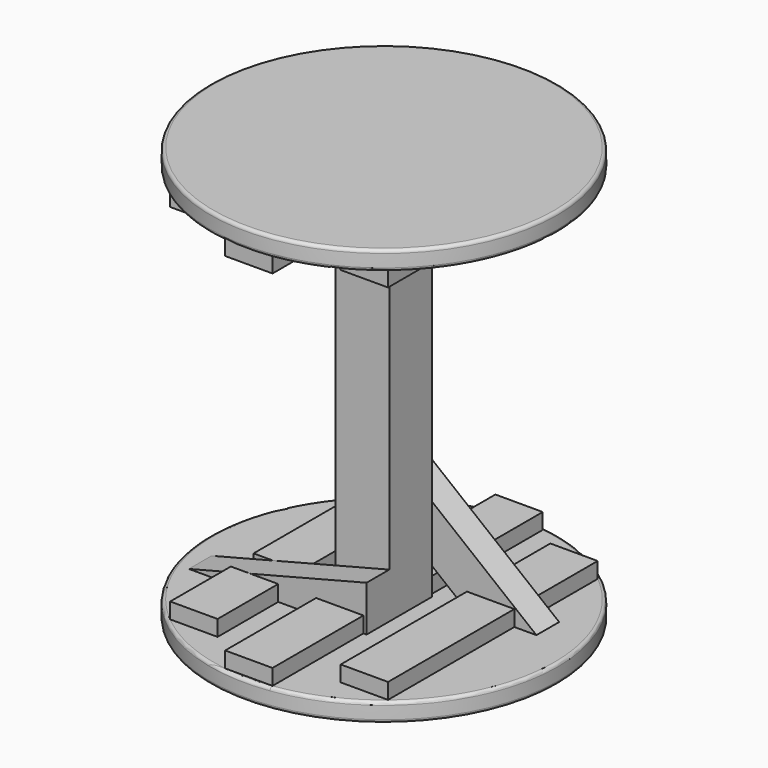
from build123d import *

# Parameters (mm, degrees)
F0_R     = 275
F1_DEPTH = 30
F2_W     = 85
F2_H     = 85
F3_DEPTH = 300
F4_W     = 75
F4_H     = 120
F4_H_2   = 250
F4_H_3   = 180
F5_DEPTH = 25
F7_DEPTH = 45
F9_DEPTH = 45


# Not quite as in the source:
# - a fillet or chamfer that OpenCascade refuses, or shapes differently, is made with other operations: its cross-section is extruded or revolved along the edge and cut away or added


with BuildPart() as f1:
    # F0 (on Top) → F1 (new body)
    with BuildSketch(Plane.XY):
        Circle(F0_R)
    extrude(amount=F1_DEPTH)

    # F2 (on face) → F3 (join)
    with BuildSketch(Plane(origin=(0, 0, 0), x_dir=(1, 0, 0), z_dir=(0, 0, -1))):
        Rectangle(F2_W, F2_H)
    extrude(amount=F3_DEPTH)

    # F4 (on face) → F5 (join)
    with BuildSketch(Plane(origin=(0, 0, 0), x_dir=(1, 0, 0), z_dir=(0, 0, -1))):
        Polygon((37.5, -267.5), (37.5, -42.5), (0, -42.5), (-37.5, -42.5), (-37.5, -267.5), (0, -267.5), align=None)
        with Locations((-135, 147.5)):
            Rectangle(F4_W, F4_H)
        with Locations((-135, -82.5)):
            Rectangle(F4_W, F4_H_2)
        with Locations((135, 82.5)):
            Rectangle(F4_W, F4_H_2)
        with Locations((135, -147.5)):
            Rectangle(F4_W, F4_H)
        with Locations((0, 177.5)):
            Rectangle(F4_W, F4_H_3)
    extrude(amount=F5_DEPTH)

    # F6 (on face) → F7 (join)
    with BuildSketch(Plane.XZ.offset(42.5)):
        Polygon((42.5, 0), (-239.0592902313, 0), (42.5, -72.2690859077), align=None)
    extrude(amount=F7_DEPTH)

    # F8 (on face) → F9 (join)
    with BuildSketch(Plane(origin=(0, 42.5, 0), x_dir=(-1, 0, 0), z_dir=(0, 1, 0))):
        Polygon((42.5, -110.4884261255), (-95.5, 0), (-207.5, 0), (42.5, -200.1601922564), align=None)
    extrude(amount=F9_DEPTH)

    # F11: fillet of radius 5 on 2 edges, made by hand

    # F11_s1 → F11_t2 (revolve, cut)
    with BuildSketch(Plane.XZ):
        with BuildLine():
            ThreePointArc((275, 25), (273.5355339059, 28.5355339059), (270, 30))
            Line((270, 30), (275, 30))
            Line((275, 30), (275, 25))
        make_face()
    revolve(axis=Axis((0, 0, 30), (0, 0, 1)), mode=Mode.SUBTRACT)


with BuildPart() as f11_tool4:
    # F11_s5 → F11_t6 (revolve)
    with BuildSketch(Plane.XZ):
        with BuildLine():
            ThreePointArc((275, 5), (273.5355339059, 1.4644660941), (270, 0))
            Line((270, 0), (275, 0))
            Line((275, 0), (275, 5))
        make_face()
    revolve(axis=Axis((0, 0, 0), (0, 0, 1)))

    split(bisect_by=Plane.YZ.offset(37.5), keep=Keep.TOP)


with BuildPart() as f1_1:
    add(f1.part)

    # F11_t3: cut F11_tool4
    add(f11_tool4.part, mode=Mode.SUBTRACT)


with BuildPart() as f11_tool9:
    # F11_s10 → F11_t11 (revolve)
    with BuildSketch(Plane.XZ):
        with BuildLine():
            ThreePointArc((275, 5), (273.5355339059, 1.4644660941), (270, 0))
            Line((270, 0), (275, 0))
            Line((275, 0), (275, 5))
        make_face()
    revolve(axis=Axis((0, 0, 0), (0, 0, 1)))

    split(bisect_by=Plane.XZ.offset(-267.5), keep=Keep.BOTTOM)


with BuildPart() as f1_2:
    add(f1_1.part)

    # F11_t8: cut F11_tool9
    add(f11_tool9.part, mode=Mode.SUBTRACT)


with BuildPart() as f11_tool14:
    # F11_s15 → F11_t16 (revolve)
    with BuildSketch(Plane.XZ):
        with BuildLine():
            ThreePointArc((275, 5), (273.5355339059, 1.4644660941), (270, 0))
            Line((270, 0), (275, 0))
            Line((275, 0), (275, 5))
        make_face()
    revolve(axis=Axis((0, 0, 0), (0, 0, 1)))

    split(bisect_by=Plane.XZ.offset(267.5), keep=Keep.TOP)


with BuildPart() as f1_3:
    add(f1_2.part)

    # F11_t13: cut F11_tool14
    add(f11_tool14.part, mode=Mode.SUBTRACT)


with BuildPart() as f11_tool19:
    # F11_s20 → F11_t21 (revolve)
    with BuildSketch(Plane.XZ):
        with BuildLine():
            ThreePointArc((275, 5), (273.5355339059, 1.4644660941), (270, 0))
            Line((270, 0), (275, 0))
            Line((275, 0), (275, 5))
        make_face()
    revolve(axis=Axis((0, 0, 0), (0, 0, 1)))

    split(bisect_by=Plane.YZ.offset(-37.5), keep=Keep.BOTTOM)


with BuildPart() as f1_4:
    add(f1_3.part)

    # F11_t18: cut F11_tool19
    add(f11_tool19.part, mode=Mode.SUBTRACT)

    # F12: F1 across plane


with BuildPart() as f1_5:
    add(f1_4.part)
    add(f1_4.part.mirror(Plane(origin=(0, 0, -300), x_dir=(1, 0, 0), z_dir=(0, 0, -1))))


solid = f1_5.part
